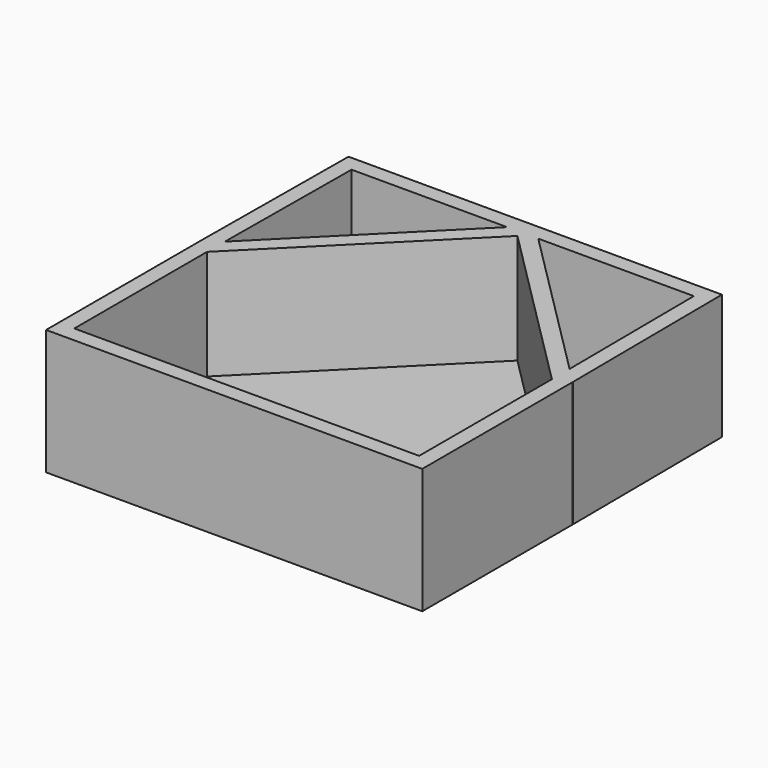
from build123d import *

# Parameters (mm, degrees)
F1_DEPTH = 50.8
F2_T     = -6.35
F4_E4_W  = 76.2411638441
F4_E4_H  = 50.8
F5_DEPTH = 6.35
F4_E3_W  = 75.6305083632
F4_E3_H  = 50.8
F6_DEPTH = 6.35


# Not quite as in the source:
# - a feature of the source that left no trace in its solid (it failed there, or was rolled back) is left out
# - a pattern or mirror of a feature is missing from the dataset's text; its kind, count and spacing are read off the source's solid


with BuildPart() as f1:
    # F0 (on Top) → F1 (new body)
    with BuildSketch(Plane.XY):
        Polygon((76.1932209134, 0), (0, 76.1944577098), (-76.1932209134, 0), (-76.1932209134, -76.1944577098), (76.1932209134, -76.1944577098), align=None)
    extrude(amount=F1_DEPTH)

    # F2
    f2_openings = [f1.faces().sort_by_distance(p)[0] for p in [
        (0, -16.932102, 50.8),
    ]]
    offset(amount=F2_T, openings=f2_openings)

    # F4_E4 (on explicit) → F5 (join)
    with BuildSketch(Plane(origin=(75.6305083632, 76.2389451265, 0), x_dir=(0.0076290083, -0.9999708987, 0), z_dir=(-0.9999708987, -0.0076290083, 0))):
        with Locations((38.120581922, 25.4)):
            Rectangle(F4_E4_W, F4_E4_H)
    f5 = extrude(amount=F5_DEPTH)

    # F5_copies: F5 across plane
    add(f5.mirror(Plane(origin=(0, 0, 0), x_dir=(0, 0, -1), z_dir=(-1, 0, 0))))

    # F4_E3 (on explicit) → F6 (join)
    with BuildSketch(Plane.XZ.offset(-76.2389451265)):
        with Locations((37.8152541816, 25.4)):
            Rectangle(F4_E3_W, F4_E3_H)
    f6 = extrude(amount=F6_DEPTH)

    # F6_copies: F6 across plane
    add(f6.mirror(Plane(origin=(0, 0, 0), x_dir=(0, 0, -1), z_dir=(-1, 0, 0))))


solid = f1.part
